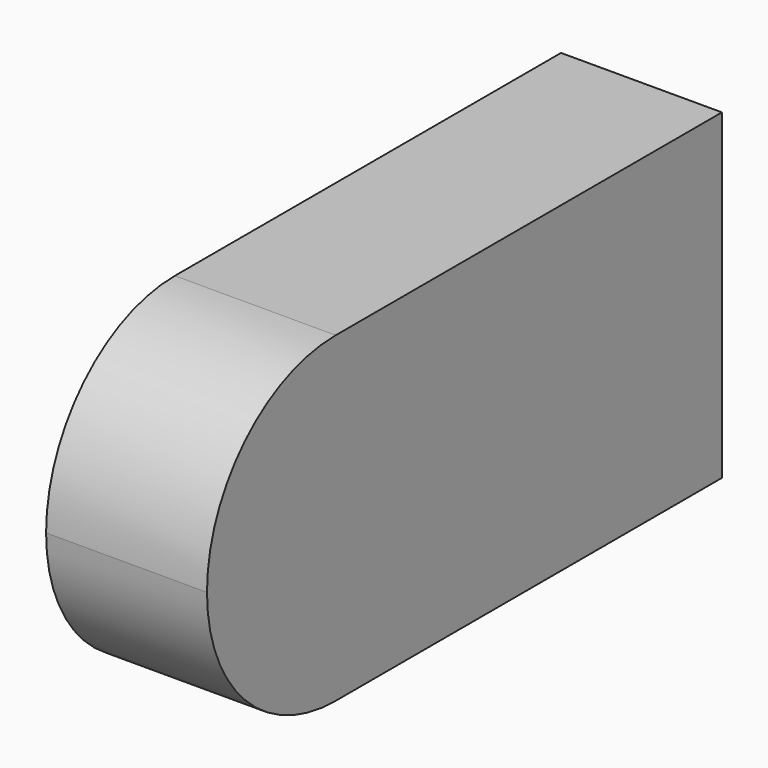
from build123d import *

# Parameters (mm, degrees)
F0_W     = 6.35
F0_H     = 12.7
F1_DEPTH = 25.4
F2_R     = 6.34999
F3_R     = 3.175
F4_DEPTH = 3.175


# Not quite as in the source:
# - a fillet or chamfer is up to 0.001 mm smaller than in the source, because OpenCascade refuses the exact size


with BuildPart() as f1:
    # F0 (on Front) → F1 (new body)
    with BuildSketch(Plane.XZ):
        Rectangle(F0_W, F0_H)
    extrude(amount=F1_DEPTH)

    # F2 (radius 6.35 in the source; OpenCascade refuses exactly that, so slightly less here)
    f2_edges = [f1.edges().sort_by_distance(p)[0] for p in [
        (0, -25.4, 6.35),
        (0, -25.4, -6.35),
    ]]
    fillet(f2_edges, radius=F2_R)

    # F3 (on face) → F4 (cut)
    with BuildSketch(Plane(origin=(-3.175, 0, 0), x_dir=(0, -1, 0), z_dir=(-1, 0, 0))):
        with Locations((19.05, 0)):
            Circle(F3_R)
    extrude(amount=-F4_DEPTH, mode=Mode.SUBTRACT)


solid = f1.part
